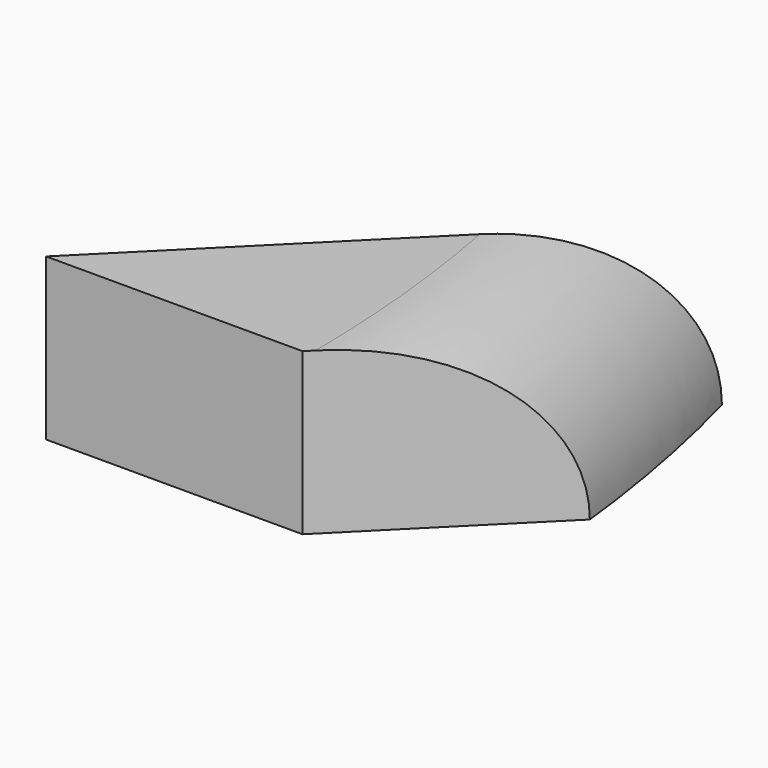
from build123d import *

# Parameters (mm, degrees)
F2_DEPTH = 25.4
F3_R     = 25.39999


# Not quite as in the source:
# - a fillet or chamfer is up to 0.001 mm smaller than in the source, because OpenCascade refuses the exact size


with BuildPart() as f2:
    # F1 (on face) → F2 (new body)
    with BuildSketch(Plane.XY):
        with BuildLine():
            Line((161.6446101792, 0), (202.0557627241, 0))
            Line((202.0557627241, 0), (227.2116647397, 25.1559020156))
            ThreePointArc((227.2116647397, 25.1559020156), (224.6556687953, 42.28227144), (220.8106438897, 59.1660337104))
            Line((220.8106438897, 59.1660337104), (161.6446101792, 0))
        make_face()
    extrude(amount=F2_DEPTH)

    # F3 (radius 25.4 in the source; OpenCascade refuses exactly that, so slightly less here)
    f3_edges = [f2.edges().sort_by_distance(p)[0] for p in [
        (224.655669, 42.282271, 25.4),
    ]]
    fillet(f3_edges, radius=F3_R)


solid = f2.part
